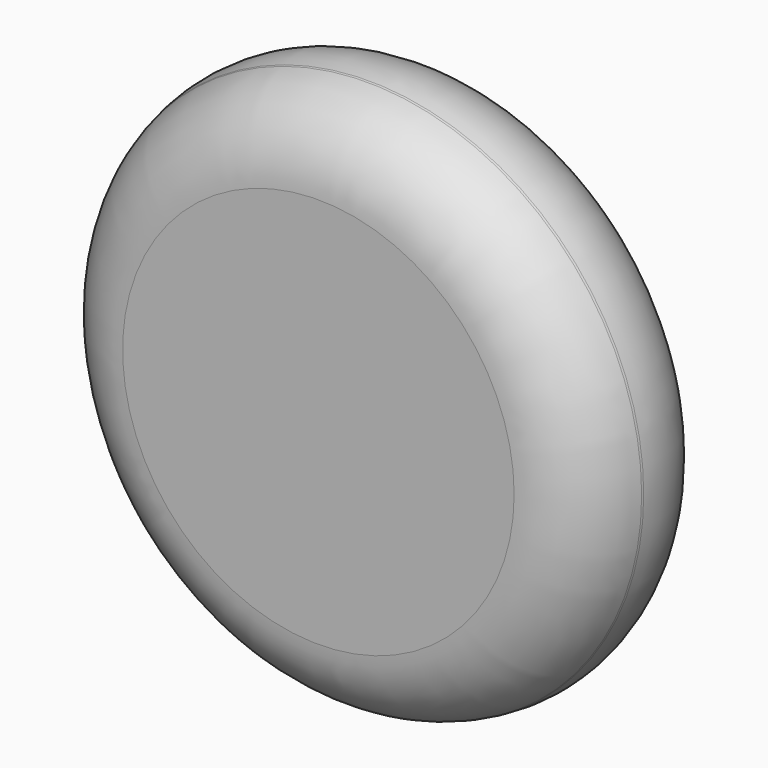
from build123d import *

# Parameters (mm, degrees)
F0_R = 40.932044689
F2_R = 35.4277651733
F4_R = 11.0387423769


with BuildPart() as f3:
    # F0 (on Front) → F3 section 0
    with BuildSketch(Plane.XZ):
        Circle(F0_R)
    # F2 (on offset) → F3 section 1
    with BuildSketch(Plane.XZ.offset(22.352)):
        Circle(F2_R)
    loft()

    # F4
    f4_edges = [f3.edges().sort_by_distance(p)[0] for p in [
        (-35.427765, -22.352, 0),
        (-40.932045, 0, 0),
        (38.179905, -11.176, 0),
    ]]
    fillet(f4_edges, radius=F4_R)


solid = f3.part
